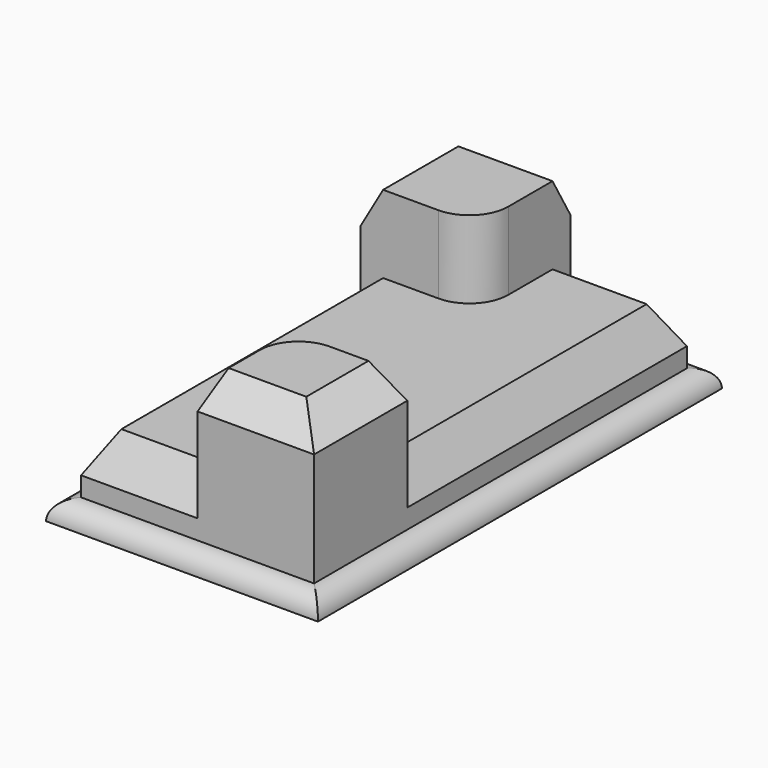
from build123d import *

# Parameters (mm, degrees)
F0_W        = 88.9
F0_H        = 165.1
F1_DEPTH    = 6.35
F2_DEPTH    = 25.4
F3_DEPTH    = 50.8
F4_C1_SIZE2 = 7.3323484187
F4_C1_SIZE  = 12.7
F4_C2_SIZE2 = 7.3323484187
F4_C2_SIZE  = 12.7
F4_C3_SIZE2 = 12.7
F4_C3_SIZE  = 7.3323484187
F4_C4_SIZE2 = 7.3323484187
F4_C4_SIZE  = 12.7
F4_C5_SIZE2 = 12.7
F4_C5_SIZE  = 7.3323484187
F4_C6_SIZE2 = 12.7
F4_C6_SIZE  = 7.3323484187
F4_C7_SIZE2 = 7.3323484187
F4_C7_SIZE  = 12.7
F4_C8_SIZE2 = 7.3323484187
F4_C8_SIZE  = 12.7
F5_R        = 6.34999


# Not quite as in the source:
# - a fillet or chamfer is up to 0.001 mm smaller than in the source, because OpenCascade refuses the exact size


with BuildPart() as f1:
    # F0 (on Top) → F1 (new body)
    with BuildSketch(Plane.XY):
        Rectangle(F0_W, F0_H)
        Polygon((0, 76.2), (38.1, 76.2), (38.1, -38.1), (38.1, -76.2), (0, -76.2), (-38.1, -76.2), (-38.1, 38.1), (-38.1, 76.2), align=None, mode=Mode.SUBTRACT)
    extrude(amount=F1_DEPTH)

    # F0 (on Top) → F2 (join)
    with BuildSketch(Plane.XY):
        with BuildLine():
            Line((38.1, -38.1), (38.1, 76.2))
            Line((38.1, 76.2), (0, 76.2))
            Line((0, 76.2), (0, 50.8))
            ThreePointArc((0, 50.8), (-3.7197438789, 41.8197438789), (-12.7, 38.1))
            Line((-12.7, 38.1), (-38.1, 38.1))
            Line((-38.1, 38.1), (-38.1, -76.2))
            Line((-38.1, -76.2), (0, -76.2))
            Line((0, -76.2), (0, -50.8))
            ThreePointArc((0, -50.8), (3.7197438789, -41.8197438789), (12.7, -38.1))
            Line((12.7, -38.1), (38.1, -38.1))
        make_face()
    extrude(amount=F2_DEPTH)

    # F0 (on Top) → F3 (join)
    with BuildSketch(Plane.XY):
        with BuildLine():
            Line((0, 50.8), (0, 76.2))
            Line((0, 76.2), (-38.1, 76.2))
            Line((-38.1, 76.2), (-38.1, 38.1))
            Line((-38.1, 38.1), (-12.7, 38.1))
            ThreePointArc((-12.7, 38.1), (-3.7197438789, 41.8197438789), (0, 50.8))
        make_face()
        with BuildLine():
            Line((38.1, -76.2), (38.1, -38.1))
            Line((38.1, -38.1), (12.7, -38.1))
            ThreePointArc((12.7, -38.1), (3.7197438789, -41.8197438789), (0, -50.8))
            Line((0, -50.8), (0, -76.2))
            Line((0, -76.2), (38.1, -76.2))
        make_face()
    extrude(amount=F3_DEPTH)

    # F4: chamfer of 12.7 x 7.3323484187 on 8 edges, made by hand

    # F4_c1
    f4_c1_edges = [f1.edges().sort_by_distance(p)[0] for p in [
        (-38.1, 57.15, 50.8),
    ]]
    f4_c1_side = f1.faces().sort_by_distance((-38.1, 57.15, 50.6533530316))[0]
    chamfer(f4_c1_edges, length=F4_C1_SIZE, length2=F4_C1_SIZE2, reference=f4_c1_side)

    # F4_c2
    f4_c2_edges = [f1.edges().sort_by_distance(p)[0] for p in [
        (-38.1, -19.05, 25.4),
    ]]
    f4_c2_side = f1.faces().sort_by_distance((-38.1, -19.05, 25.2533530316))[0]
    chamfer(f4_c2_edges, length=F4_C2_SIZE, length2=F4_C2_SIZE2, reference=f4_c2_side)

    # F4_c3
    f4_c3_edges = [f1.edges().sort_by_distance(p)[0] for p in [
        (38.1, 19.05, 25.4),
    ]]
    f4_c3_side = f1.faces().sort_by_distance((37.9533530316, 19.05, 25.4))[0]
    chamfer(f4_c3_edges, length=F4_C3_SIZE, length2=F4_C3_SIZE2, reference=f4_c3_side)

    # F4_c4
    f4_c4_edges = [f1.edges().sort_by_distance(p)[0] for p in [
        (15.3838257906, 76.2, 25.4),
    ]]
    f4_c4_side = f1.faces().sort_by_distance((15.3838257906, 76.2, 25.2533530316))[0]
    chamfer(f4_c4_edges, length=F4_C4_SIZE, length2=F4_C4_SIZE2, reference=f4_c4_side)

    # F4_c5
    f4_c5_edges = [f1.edges().sort_by_distance(p)[0] for p in [
        (-15.3838257906, -76.2, 25.4),
    ]]
    f4_c5_side = f1.faces().sort_by_distance((-15.3838257906, -76.0533530316, 25.4))[0]
    chamfer(f4_c5_edges, length=F4_C5_SIZE, length2=F4_C5_SIZE2, reference=f4_c5_side)

    # F4_c6
    f4_c6_edges = [f1.edges().sort_by_distance(p)[0] for p in [
        (19.05, -76.2, 50.8),
    ]]
    f4_c6_side = f1.faces().sort_by_distance((19.05, -76.2, 50.6533530316))[0]
    chamfer(f4_c6_edges, length=F4_C6_SIZE, length2=F4_C6_SIZE2, reference=f4_c6_side)

    # F4_c7
    f4_c7_edges = [f1.edges().sort_by_distance(p)[0] for p in [
        (38.1, -50.8, 50.8),
    ]]
    f4_c7_side = f1.faces().sort_by_distance((37.9533530316, -50.8, 50.8))[0]
    chamfer(f4_c7_edges, length=F4_C7_SIZE, length2=F4_C7_SIZE2, reference=f4_c7_side)

    # F4_c8
    f4_c8_edges = [f1.edges().sort_by_distance(p)[0] for p in [
        (-15.3838257906, 76.2, 50.8),
    ]]
    f4_c8_side = f1.faces().sort_by_distance((-15.3838257906, 76.2, 50.6533530316))[0]
    chamfer(f4_c8_edges, length=F4_C8_SIZE, length2=F4_C8_SIZE2, reference=f4_c8_side)

    # F5 (radius 6.35 in the source; OpenCascade refuses exactly that, so slightly less here)
    f5_edges = [f1.edges().sort_by_distance(p)[0] for p in [
        (0, -82.55, 6.35),
        (-44.45, 0, 6.35),
        (44.45, 0, 6.35),
        (0, 82.55, 6.35),
    ]]
    fillet(f5_edges, radius=F5_R)


solid = f1.part
